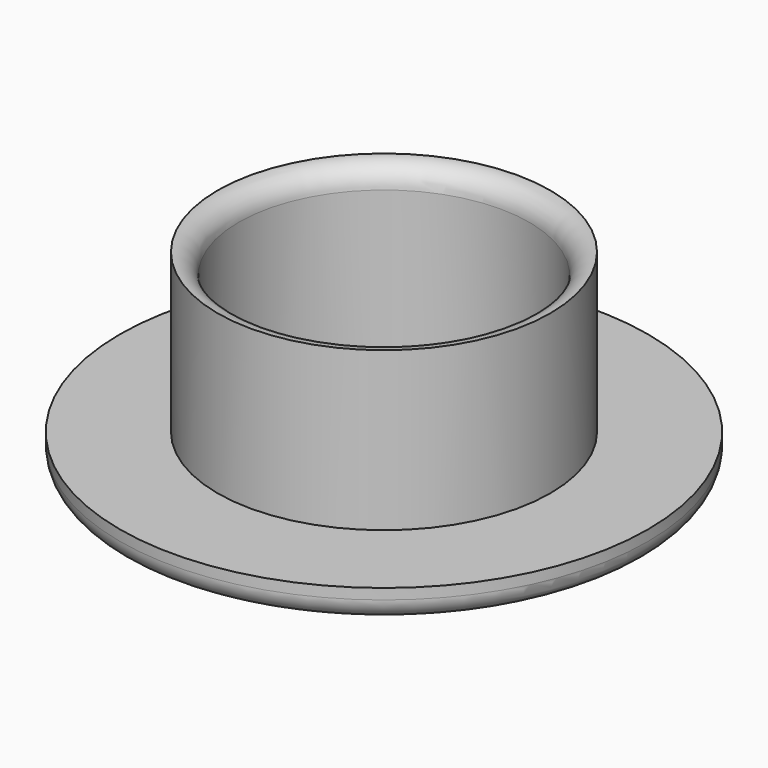
from build123d import *

# Parameters (mm, degrees)
F0_R     = 25
F1_DEPTH = 3
F2_R     = 15.75
F3_DEPTH = 15
F4_R     = 13.75
F5_DEPTH = 18
F6_R     = 1.99999


# Not quite as in the source:
# - a fillet or chamfer is up to 0.001 mm smaller than in the source, because OpenCascade refuses the exact size


with BuildPart() as f1:
    # F0 (on Top) → F1 (new body)
    with BuildSketch(Plane.XY):
        Circle(F0_R)
    extrude(amount=F1_DEPTH)

    # F2 (on face) → F3 (join)
    with BuildSketch(Plane.XY.offset(3)):
        Circle(F2_R)
    extrude(amount=F3_DEPTH)

    # F4 (on face) → F5 (cut, through all)
    with BuildSketch(Plane.XY.offset(18)):
        Circle(F4_R)
    extrude(amount=-F5_DEPTH, mode=Mode.SUBTRACT)

    # F6 (radius 2 in the source; OpenCascade refuses exactly that, so slightly less here)
    f6_edges = [f1.edges().sort_by_distance(p)[0] for p in [
        (-25, 0, 0),
        (-13.75, 0, 0),
        (-13.75, 0, 18),
    ]]
    fillet(f6_edges, radius=F6_R)


solid = f1.part
